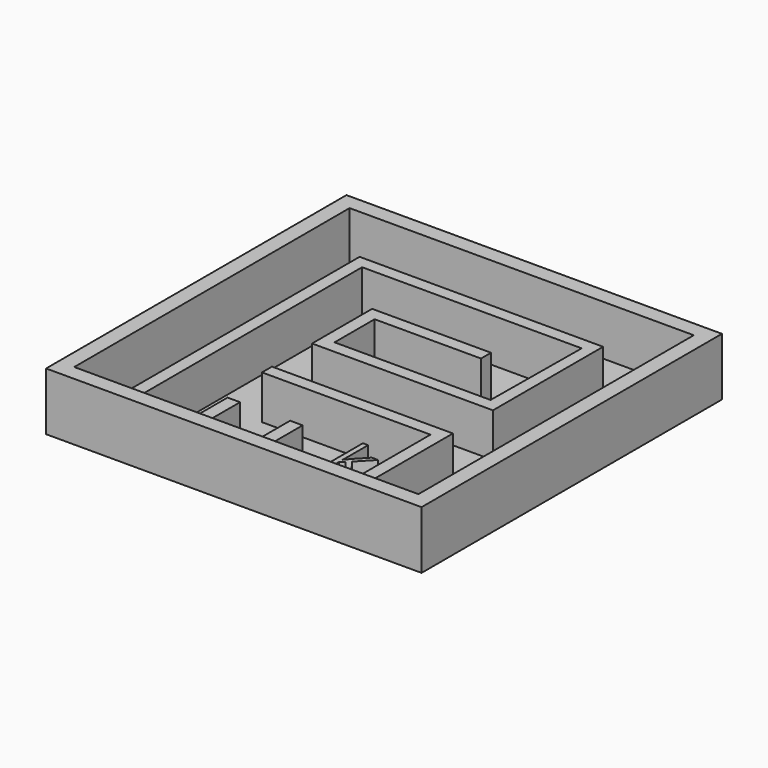
from build123d import *

# Parameters (mm, degrees)
F0_W         = 38.1
F0_H         = 38.1
F1_DEPTH     = 0.79375
F2_W         = 38.1
F2_H         = 38.1
F2_W_2       = 34.925
F2_H_2       = 34.925
F3_DEPTH     = 5.08
F4_W         = 1.27
F4_H         = 4.445
F4_TEXT_SIZE = 6.6145833333
F5_DEPTH     = 4.445
F6_R         = 1.27
F7_DEPTH     = 0.396875


# Not quite as in the source:
# - Text() gives the source's letters only with a copy of the font that has no kerning and outlines rounded to 1/6400 em; it was checked with that copy


with BuildPart() as f1:
    # F0 (on Top) → F1 (new body)
    with BuildSketch(Plane.XY):
        with Locations((-0.2397205681, 3.2357953655)):
            Rectangle(F0_W, F0_H)
    extrude(amount=F1_DEPTH)

    # F2 (on face) → F3 (join)
    with BuildSketch(Plane.XY.offset(0.79375)):
        with Locations((-0.2397205681, 3.2357953655)):
            Rectangle(F2_W, F2_H)
        with Locations((-0.2397205681, 3.2357953655)):
            Rectangle(F2_W_2, F2_H_2, mode=Mode.SUBTRACT)
    extrude(amount=F3_DEPTH)

    # F4 (on face) → F5 (join)
    with BuildSketch(Plane.XY.offset(0.79375)):
        Polygon((-12.6222205681, 15.6182953655), (-12.6222205681, -14.2267046345), (-11.3522205681, -14.2267046345), (-11.3522205681, 14.3482953655), (-11.3522205681, 15.6182953655), align=None)
        Polygon((-11.3522205681, 15.6182953655), (-11.3522205681, 14.3482953655), (10.9304172235, 14.3482953655), (10.8270431612, 2.9182953655), (-5.0022205681, 2.9182953655), (-5.0022205681, 7.9982953655), (5.7927794319, 7.9982953655), (5.7927794319, 9.2682953655), (-5.0022205681, 9.2682953655), (-6.2722205681, 9.2682953655), (-6.2722205681, 2.9182953655), (-6.2722205681, 1.6482953655), (10.8155571542, 1.6482953655), (12.0855571542, 1.6482953655), (12.0855571542, 15.6182953655), align=None)
        Polygon((12.0855571542, -14.2267046345), (12.0855571542, -3.4317046345), (10.8270431612, -3.4317046345), (-6.2722205681, -3.4317046345), (-6.2722205681, -4.7017046345), (10.8270431612, -4.7017046345), (10.8270431612, -14.2267046345), align=None)
        with Locations((1.2817859997, -12.0042046345)):
            Rectangle(F4_W, F4_H)
        with Locations((-5.0682140003, -12.0042046345)):
            Rectangle(F4_W, F4_H)
        with Locations((6.9967859997, -14.2267046345)):
            Text('k', F4_TEXT_SIZE, font='Open Sans', text_align=(TextAlign.LEFT, TextAlign.BOTTOM))
    extrude(amount=F5_DEPTH)

    # F6 (on face) → F7 (cut)
    with BuildSketch(Plane.XY.offset(0.79375)):
        with Locations((-15.1622205681, -11.369129098)):
            Circle(F6_R)
        with Locations((4.7410063773, -11.3771231845)):
            Circle(F6_R)
    extrude(amount=-F7_DEPTH, mode=Mode.SUBTRACT)


solid = f1.part
